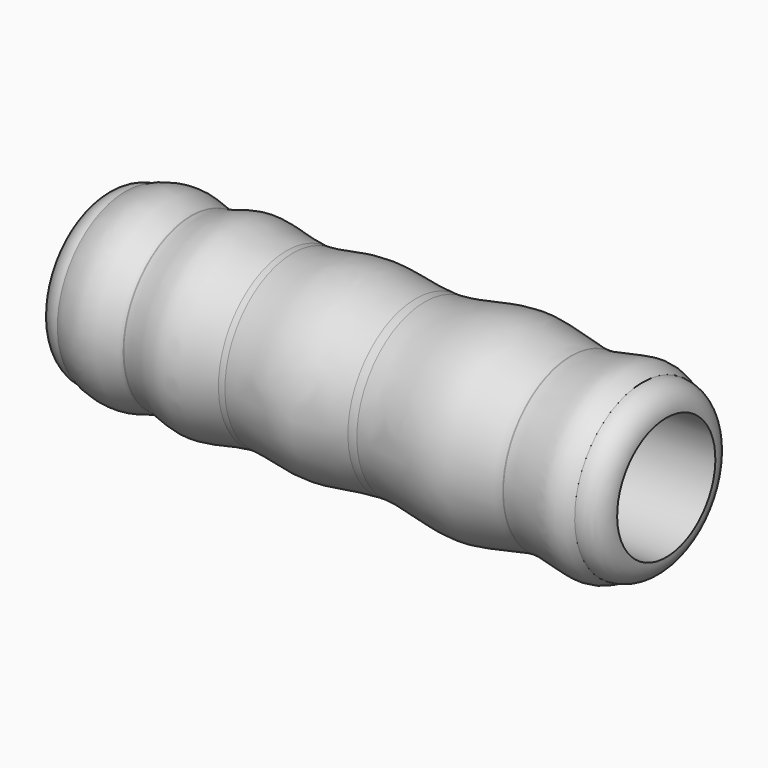
from build123d import *


with BuildPart() as f1:
    # F0 (on Front) → F1 (revolve)
    with BuildSketch(Plane.XZ):
        with BuildLine():
            Line((-75.6412, 16.51), (76.2, 16.51))
            ThreePointArc((76.2, 16.51), (74.3401280605, 21.0001280605), (69.85, 22.86))
            Line((69.85, 22.86), (50.7000796497, 22.86))
            add(Edge.make_bspline(
                [(50.5058497264, 22.86), (50.5706057369, 22.8596754076), (50.6353489577, 22.8596730925), (50.7000796497, 22.86)],
                knots=[0.8323923136, 0.8323923136, 0.8323923136, 0.8323923136, 0.8336677213, 0.8336677213, 0.8336677213, 0.8336677213], degree=3))
            Line((50.5058497264, 22.86), (11.2541196868, 22.86))
            add(Edge.make_bspline(
                [(8.8545044549, 22.86), (9.654443387, 22.8335928328), (10.4546819055, 22.8313514547), (11.2541196868, 22.86)],
                knots=[0.5777964989, 0.5777964989, 0.5777964989, 0.5777964989, 0.5916792469, 0.5916792469, 0.5916792469, 0.5916792469], degree=3))
            Line((8.8545044549, 22.86), (-24.2349496389, 22.86))
            add(Edge.make_bspline(
                [(-25.9719379246, 22.86), (-25.3904076002, 22.836978978), (-24.8117447825, 22.8386038349), (-24.2349496389, 22.86)],
                knots=[0.357508186, 0.357508186, 0.357508186, 0.357508186, 0.3692777281, 0.3692777281, 0.3692777281, 0.3692777281], degree=3))
            Line((-25.9719379246, 22.86), (-51.4154396951, 22.86))
            add(Edge.make_bspline(
                [(-51.6103026405, 22.86), (-51.5454772703, 22.8591105526), (-51.4805272698, 22.8590976396), (-51.4154396951, 22.86)],
                knots=[0.1618012553, 0.1618012553, 0.1618012553, 0.1618012553, 0.1637198302, 0.1637198302, 0.1637198302, 0.1637198302], degree=3))
            Line((-51.6103026405, 22.86), (-69.2912, 22.86))
            ThreePointArc((-69.2912, 22.86), (-73.7813280605, 21.0001280605), (-75.6412, 16.51))
        make_face()
        with BuildLine():
            Line((50.7000796497, 22.86), (69.85, 22.86))
            add(Edge.make_bspline(
                [(50.7000796497, 22.86), (55.8146208152, 22.8858298184), (64.1273713818, 26.3209146353), (68.2820749394, 23.807391724), (69.85, 22.86)],
                knots=[0.8336677213, 0.8336677213, 0.8336677213, 0.8336677213, 0.9344410153, 1, 1, 1, 1], degree=3))
        make_face()
        with BuildLine():
            add(Edge.make_bspline(
                [(-69.2912, 22.86), (-67.0878619126, 24.1767972382), (-59.2480814587, 25.9249777514), (-54.201168592, 22.8955484125), (-51.6103026405, 22.86)],
                knots=[0, 0, 0, 0, 0.0851218586, 0.1618012553, 0.1618012553, 0.1618012553, 0.1618012553], degree=3))
            Line((-69.2912, 22.86), (-51.6103026405, 22.86))
        make_face()
        with BuildLine():
            Line((11.2541196868, 22.86), (50.5058497264, 22.86))
            add(Edge.make_bspline(
                [(11.2541196868, 22.86), (18.4729734076, 23.1186938759), (32.2090595343, 28.4518581182), (44.6490527547, 22.8893574606), (50.5058497264, 22.86)],
                knots=[0.5916792469, 0.5916792469, 0.5916792469, 0.5916792469, 0.717039256, 0.8323923136, 0.8323923136, 0.8323923136, 0.8323923136], degree=3))
        make_face()
        with BuildLine():
            add(Edge.make_bspline(
                [(-51.4154396951, 22.86), (-48.4856501908, 22.900617985), (-41.2858930569, 27.153149401), (-31.279904219, 23.0701262886), (-25.9719379246, 22.86)],
                knots=[0.1637198302, 0.1637198302, 0.1637198302, 0.1637198302, 0.2500807141, 0.357508186, 0.357508186, 0.357508186, 0.357508186], degree=3))
            Line((-51.4154396951, 22.86), (-25.9719379246, 22.86))
        make_face()
        with BuildLine():
            Line((-24.2349496389, 22.86), (8.8545044549, 22.86))
            add(Edge.make_bspline(
                [(-24.2349496389, 22.86), (-19.4137140956, 23.0388433081), (-9.4713243481, 26.34582534), (2.5080525383, 23.0695057634), (8.8545044549, 22.86)],
                knots=[0.3692777281, 0.3692777281, 0.3692777281, 0.3692777281, 0.4676553499, 0.5777964989, 0.5777964989, 0.5777964989, 0.5777964989], degree=3))
        make_face()
    revolve(axis=Axis((38.1, 0, 0), (1, 0, 0)))


solid = f1.part
